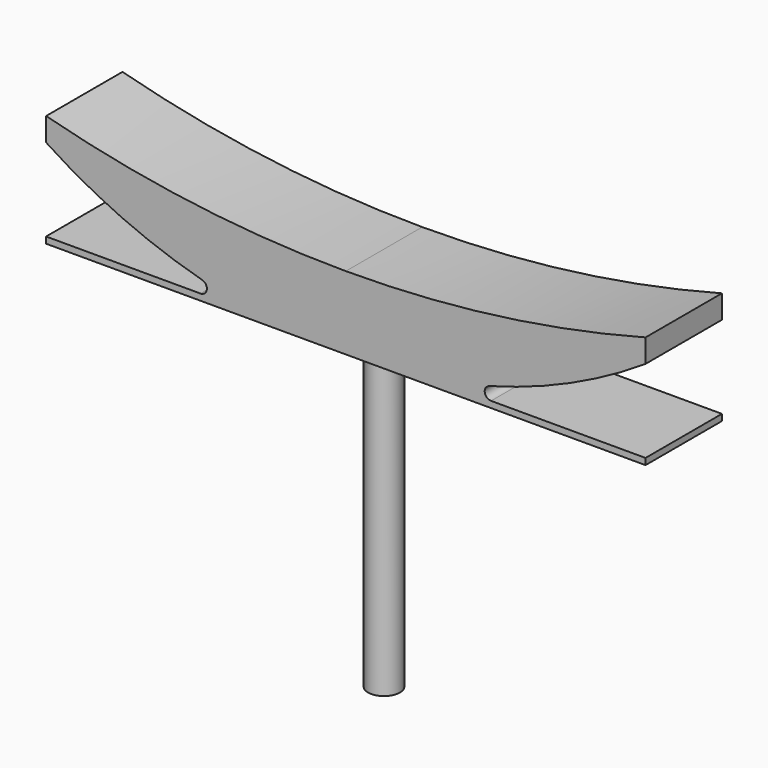
from build123d import *

# Parameters (mm, degrees)
F0_R     = 1.905
F1_DEPTH = 38.1
F2_W     = 71.755
F2_H     = 11.43
F2_R     = 1.905
F3_DEPTH = 0.762
F5_DEPTH = 11.43
F6_R     = 0.762


# Not quite as in the source:
# - a feature names something its author has since deleted; it is built from what else it names


with BuildPart() as f1:
    # F0 (on Top) → F1 (new body)
    with BuildSketch(Plane.XY):
        Circle(F0_R)
    extrude(amount=F1_DEPTH)

    # F2 (on face) → F3 (join)
    with BuildSketch(Plane.XY.offset(38.1)):
        Rectangle(F2_W, F2_H)
        Circle(F2_R, mode=Mode.SUBTRACT)
    extrude(amount=-F3_DEPTH)

    # F4 (on face) → F5 (join, through all)
    with BuildSketch(Plane.XZ.offset(5.715)):
        with BuildLine():
            ThreePointArc((0, 46.1144251321), (-18.0910863279, 47.2907715726), (-35.8775, 50.8))
            Line((-35.8775, 50.8), (-35.8775, 48.0069763479))
            ThreePointArc((-35.8775, 48.0069763479), (-23.5669827894, 41.6891623658), (-10.2035430744, 38.1))
            Line((-10.2035430744, 38.1), (0, 38.1))
            Line((0, 38.1), (0, 46.1144251321))
        make_face()
        with BuildLine():
            ThreePointArc((35.8775, 50.8), (18.0910863279, 47.2907715726), (0, 46.1144251321))
            Line((0, 46.1144251321), (0, 38.1))
            Line((0, 38.1), (10.2035430744, 38.1))
            ThreePointArc((10.2035430744, 38.1), (23.5669827894, 41.6891623658), (35.8775, 48.0069763479))
            Line((35.8775, 48.0069763479), (35.8775, 50.8))
        make_face()
    extrude(amount=-F5_DEPTH)

    # F6
    f6_edges = [f1.edges().sort_by_distance(p)[0] for p in [
        (10.203543, 0, 38.1),
        (-10.203543, 0, 38.1),
    ]]
    fillet(f6_edges, radius=F6_R)


solid = f1.part
